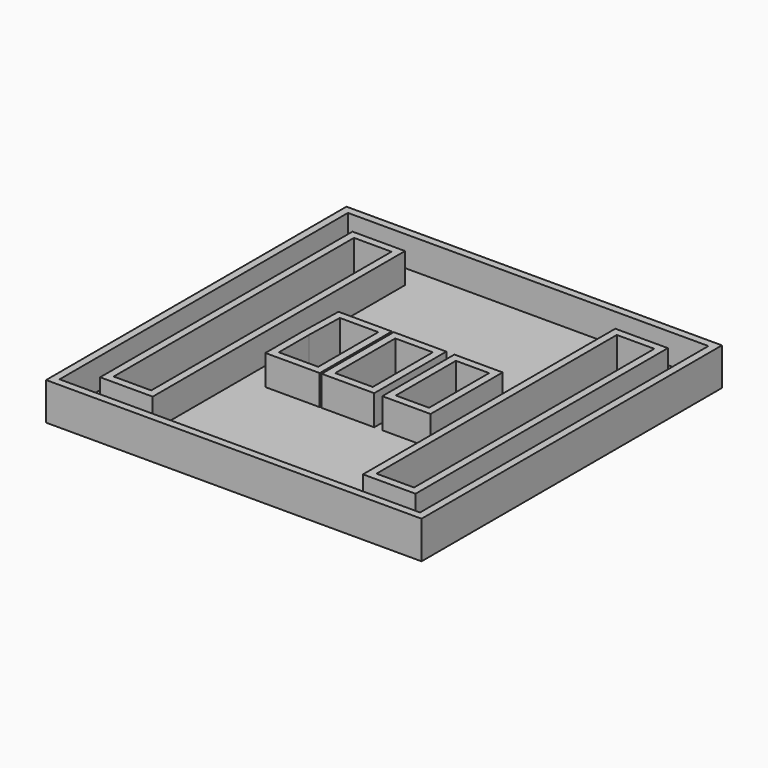
from build123d import *

# Parameters (mm, degrees)
F0_W     = 127
F0_H     = 127
F0_W_2   = 12.7
F0_H_2   = 101.6
F1_DEPTH = 12.7
F2_T     = -2.54


with BuildPart() as f1:
    # F0 (on Top) → F1 (new body)
    with BuildSketch(Plane.XY):
        with Locations((-24.9704163089, 19.614642486)):
            Rectangle(F0_W, F0_H)
        with Locations((-69.4204163089, 19.614642486)):
            Rectangle(F0_W_2, F0_H_2, mode=Mode.SUBTRACT)
        Polygon((-50.3704163089, 6.914642486), (-50.3704163089, 19.614642486), (-50.0745723798, 32.314642486), (-37.0573314681, 32.314642486), (-37.0573314681, 6.914642486), align=None, mode=Mode.SUBTRACT)
        Polygon((-31.3204163089, 32.314642486), (-24.9704163089, 32.314642486), (-18.6204163089, 32.314642486), (-18.6204163089, 6.914642486), (-31.3204163089, 6.914642486), align=None, mode=Mode.SUBTRACT)
        Polygon((0.4295836911, 32.314642486), (0.4295836911, 19.614642486), (0.4295836911, 6.914642486), (-10.8125778138, 6.914642486), (-10.8125778138, 32.314642486), align=None, mode=Mode.SUBTRACT)
        with Locations((19.4795836911, 19.614642486)):
            Rectangle(F0_W_2, F0_H_2, mode=Mode.SUBTRACT)
    extrude(amount=F1_DEPTH)

    # F2
    f2_openings = [f1.faces().sort_by_distance(p)[0] for p in [
        (36.733532, 19.614642, 12.7),
    ]]
    offset(amount=F2_T, openings=f2_openings, kind=Kind.INTERSECTION)


solid = f1.part
